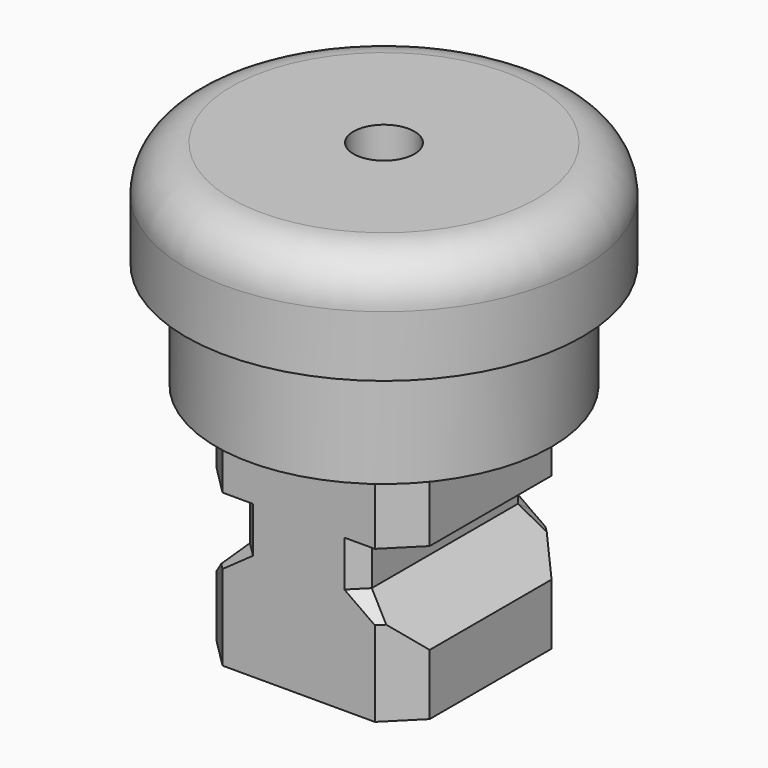
from build123d import *

# Parameters (mm, degrees)
F3_DEPTH     = 3.5
F4_SIZE      = 1
F5_SIZE      = 0.5
F6_T4_DEPTH  = 8.4221557451
F6_T11_DEPTH = 13.7150489639
F6_T21_DEPTH = 8.4221557451
F6_T28_DEPTH = 8.4221557451
F6_T35_DEPTH = 13.7150489639
F6_T45_DEPTH = 8.4221557451
F7_R         = 1.5
F8_R         = 1
F9_DEPTH     = 25


# Not quite as in the source:
# - a fillet or chamfer that OpenCascade refuses, or shapes differently, is made with other operations: its cross-section is extruded or revolved along the edge and cut away or added


with BuildPart() as f1:
    # F0 (on Front) → F1 (revolve)
    with BuildSketch(Plane.XZ):
        Polygon((0, 7), (0, 0), (5.5, 0), (5.5, 3.5), (6.5, 3.5), (6.5, 7), align=None)
    revolve(axis=Axis((0, 0, 5.0261294236), (0, 0, 1)))

    # F2 (on Front) → F3 (join, symmetric)
    with BuildSketch(Plane.XZ):
        Polygon((3.5, 0), (-3.5, 0), (-3.5, -2.5), (-2, -2.5), (-2, -5.5), (-3.5, -5.5), (-3.5, -7.5), (3.5, -7.5), (3.5, -5.5), (2, -5.5), (2, -2.5), (3.5, -2.5), align=None)
    extrude(amount=F3_DEPTH, both=True)

    # F4
    f4_edges = [f1.edges().sort_by_distance(p)[0] for p in [
        (3.5, -3.5, -1.25),
        (3.5, 3.5, -1.25),
        (-3.5, 3.5, -1.25),
        (-3.5, -3.5, -1.25),
        (-3.5, -3.5, -6.5),
        (3.5, -3.5, -6.5),
        (-3.5, 3.5, -6.5),
        (3.5, 3.5, -6.5),
    ]]
    chamfer(f4_edges, length=F4_SIZE)

    # F5
    f5_edges = [f1.edges().sort_by_distance(p)[0] for p in [
        (2, -3.5, -4),
        (-2, -3.5, -4),
        (-2, 3.5, -4),
        (2, 3.5, -4),
    ]]
    chamfer(f5_edges, length=F5_SIZE)

    # F6: chamfer of 1.5 on 6 edges, made by hand


with BuildPart() as f6_tool2:
    # F6_s3 → F6_t4 (new body)
    with BuildSketch(Plane(origin=(3.7276817198, -3.7276817198, 0), x_dir=(0, 0, 1), z_dir=(-0.7071067812, 0.7071067812, 0))):
        Polygon((-5.5, -5.0355339059), (-4, -3.5355339059), (-5.5, -3.5355339059), align=None)
    extrude(amount=F6_T4_DEPTH)

    split(bisect_by=Plane.XZ.offset(3.5), keep=Keep.BOTTOM)

    split(bisect_by=Plane(origin=(-3, -3, 0), x_dir=(0, 0, 1), z_dir=(0.7071067812, 0.7071067812, 0)), keep=Keep.TOP)

    split(bisect_by=Plane(origin=(1, 0, -1), x_dir=(0, 1, 0), z_dir=(0.7071067812, 0, -0.7071067812)), keep=Keep.TOP)


with BuildPart() as f1_1:
    add(f1.part)

    # F6_t1: union F6_tool2
    add(f6_tool2.part)


with BuildPart() as f6_tool9:
    # F6_s10 → F6_t11 (new body)
    with BuildSketch(Plane.XZ.offset(-6.8575244819)):
        Polygon((-3.5, -5.5), (-2, -4), (-2, -5.5), align=None)
    extrude(amount=F6_T11_DEPTH)

    split(bisect_by=Plane.XZ.offset(3.5), keep=Keep.BOTTOM)

    split(bisect_by=Plane(origin=(-3, -3, 0), x_dir=(0, 0, 1), z_dir=(0.7071067812, 0.7071067812, 0)), keep=Keep.TOP)

    split(bisect_by=Plane.XZ.offset(-3.5), keep=Keep.TOP)

    split(bisect_by=Plane(origin=(-3, 3, 0), x_dir=(0, 0, 1), z_dir=(0.7071067812, -0.7071067812, 0)), keep=Keep.TOP)

    split(bisect_by=Plane(origin=(0.1642135624, -0.1642135624, -0.232233047), x_dir=(0.7071067812, 0.7071067812, 0), z_dir=(0.5, -0.5, -0.7071067812)), keep=Keep.TOP)

    split(bisect_by=Plane(origin=(0.1642135624, 0.1642135624, -0.232233047), x_dir=(-0.7071067812, 0.7071067812, 0), z_dir=(0.5, 0.5, -0.7071067812)), keep=Keep.TOP)


with BuildPart() as f1_2:
    add(f1_1.part)

    # F6_t8: union F6_tool9
    add(f6_tool9.part)


with BuildPart() as f6_tool19:
    # F6_s20 → F6_t21 (new body)
    with BuildSketch(Plane(origin=(3.7276817198, 3.7276817198, 0), x_dir=(0, 0, 1), z_dir=(-0.7071067812, -0.7071067812, 0))):
        Polygon((-5.5, 5.0355339059), (-4, 3.5355339059), (-5.5, 3.5355339059), align=None)
    extrude(amount=F6_T21_DEPTH)

    split(bisect_by=Plane.XZ.offset(-3.5), keep=Keep.TOP)

    split(bisect_by=Plane(origin=(-3, 3, 0), x_dir=(0, 0, 1), z_dir=(0.7071067812, -0.7071067812, 0)), keep=Keep.TOP)

    split(bisect_by=Plane(origin=(1, 0, -1), x_dir=(0, 1, 0), z_dir=(0.7071067812, 0, -0.7071067812)), keep=Keep.TOP)


with BuildPart() as f1_3:
    add(f1_2.part)

    # F6_t18: union F6_tool19
    add(f6_tool19.part)


with BuildPart() as f6_tool26:
    # F6_s27 → F6_t28 (new body)
    with BuildSketch(Plane(origin=(-3.7276817198, -3.7276817198, 0), x_dir=(0, 0, 1), z_dir=(0.7071067812, 0.7071067812, 0))):
        Polygon((-5.5, 5.0355339059), (-4, 3.5355339059), (-5.5, 3.5355339059), align=None)
    extrude(amount=F6_T28_DEPTH)

    split(bisect_by=Plane.XZ.offset(3.5), keep=Keep.BOTTOM)

    split(bisect_by=Plane(origin=(3, -3, 0), x_dir=(0, 0, 1), z_dir=(-0.7071067812, 0.7071067812, 0)), keep=Keep.TOP)

    split(bisect_by=Plane(origin=(-1, 0, -1), x_dir=(0, 1, 0), z_dir=(-0.7071067812, 0, -0.7071067812)), keep=Keep.TOP)


with BuildPart() as f1_4:
    add(f1_3.part)

    # F6_t25: union F6_tool26
    add(f6_tool26.part)


with BuildPart() as f6_tool33:
    # F6_s34 → F6_t35 (new body)
    with BuildSketch(Plane.XZ.offset(-6.8575244819)):
        Polygon((3.5, -5.5), (2, -4), (2, -5.5), align=None)
    extrude(amount=F6_T35_DEPTH)

    split(bisect_by=Plane.XZ.offset(3.5), keep=Keep.BOTTOM)

    split(bisect_by=Plane(origin=(3, -3, 0), x_dir=(0, 0, 1), z_dir=(-0.7071067812, 0.7071067812, 0)), keep=Keep.TOP)

    split(bisect_by=Plane.XZ.offset(-3.5), keep=Keep.TOP)

    split(bisect_by=Plane(origin=(3, 3, 0), x_dir=(0, 0, 1), z_dir=(-0.7071067812, -0.7071067812, 0)), keep=Keep.TOP)

    split(bisect_by=Plane(origin=(-0.1642135624, -0.1642135624, -0.232233047), x_dir=(0.7071067812, -0.7071067812, 0), z_dir=(-0.5, -0.5, -0.7071067812)), keep=Keep.TOP)

    split(bisect_by=Plane(origin=(-0.1642135624, 0.1642135624, -0.232233047), x_dir=(-0.7071067812, -0.7071067812, 0), z_dir=(-0.5, 0.5, -0.7071067812)), keep=Keep.TOP)


with BuildPart() as f1_5:
    add(f1_4.part)

    # F6_t32: union F6_tool33
    add(f6_tool33.part)


with BuildPart() as f6_tool43:
    # F6_s44 → F6_t45 (new body)
    with BuildSketch(Plane(origin=(-3.7276817198, 3.7276817198, 0), x_dir=(0, 0, 1), z_dir=(0.7071067812, -0.7071067812, 0))):
        Polygon((-5.5, -5.0355339059), (-4, -3.5355339059), (-5.5, -3.5355339059), align=None)
    extrude(amount=F6_T45_DEPTH)

    split(bisect_by=Plane.XZ.offset(-3.5), keep=Keep.TOP)

    split(bisect_by=Plane(origin=(3, 3, 0), x_dir=(0, 0, 1), z_dir=(-0.7071067812, -0.7071067812, 0)), keep=Keep.TOP)

    split(bisect_by=Plane(origin=(-1, 0, -1), x_dir=(0, 1, 0), z_dir=(-0.7071067812, 0, -0.7071067812)), keep=Keep.TOP)


with BuildPart() as f1_6:
    add(f1_5.part)

    # F6_t42: union F6_tool43
    add(f6_tool43.part)

    # F7
    f7_edges = [f1_6.edges().sort_by_distance(p)[0] for p in [
        (-6.5, 0, 7),
    ]]
    fillet(f7_edges, radius=F7_R)

    # F8 (on face) → F9 (cut)
    with BuildSketch(Plane(origin=(0, 0, -7.5), x_dir=(1, 0, 0), z_dir=(0, 0, -1))):
        Circle(F8_R)
    extrude(amount=-F9_DEPTH, mode=Mode.SUBTRACT)


solid = f1_6.part
